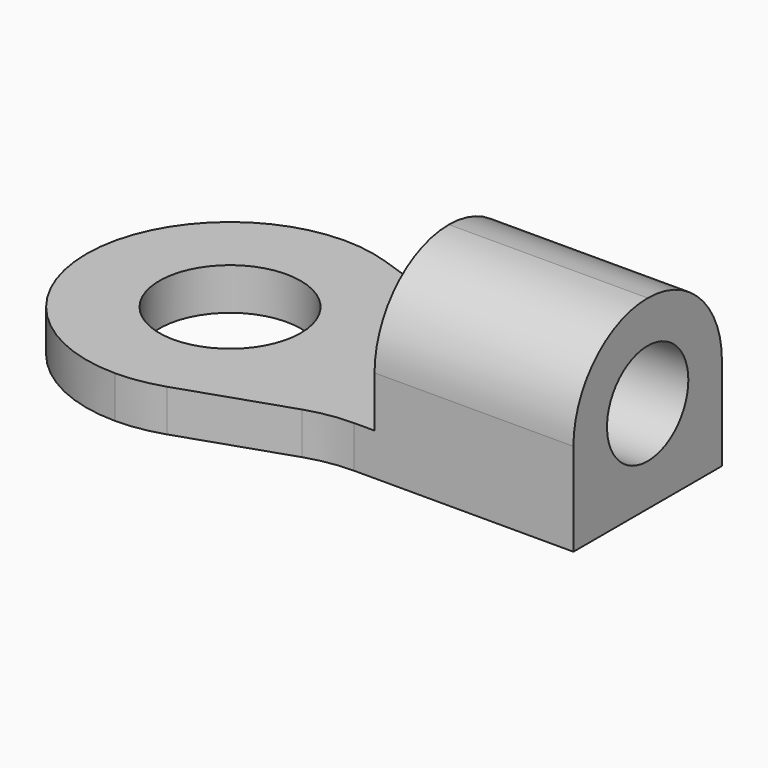
from build123d import *

# Parameters (mm, degrees)
F0_R     = 1.6
F1_DEPTH = 0.95
F2_W     = 4.5
F2_H     = 4.2
F3_DEPTH = 3.25
F4_R     = 2.09999
F5_R     = 1.15
F6_DEPTH = 25


# Not quite as in the source:
# - a fillet or chamfer is up to 0.001 mm smaller than in the source, because OpenCascade refuses the exact size


with BuildPart() as f1:
    # F0 (on Top) → F1 (new body)
    with BuildSketch(Plane.XY):
        with BuildLine():
            Line((7.7320977576, 1.15), (12.7, 1.15))
            Line((12.7, 1.15), (12.7, 5.35))
            Line((12.7, 5.35), (8.2, 5.35))
            Line((8.2, 5.35), (7.7320977576, 5.35))
            ThreePointArc((7.7320977576, 5.35), (7.2069912058, 5.3927015871), (6.6956833513, 5.5196842405))
            Line((6.6956833513, 5.5196842405), (4.2864144063, 6.3303157595))
            ThreePointArc((4.2864144063, 6.3303157595), (3.7751065518, 6.4572984129), (3.25, 6.5))
            ThreePointArc((3.25, 6.5), (0.9519029611, 5.5480970389), (0, 3.25))
            ThreePointArc((0, 3.25), (0.9519029611, 0.9519029611), (3.25, 0))
            ThreePointArc((3.25, 0), (3.7751065518, 0.0427015871), (4.2864144063, 0.1696842405))
            Line((4.2864144063, 0.1696842405), (6.6956833513, 0.9803157595))
            ThreePointArc((6.6956833513, 0.9803157595), (7.2069912058, 1.1072984129), (7.7320977576, 1.15))
        make_face()
        with Locations((3.25, 3.25)):
            Circle(F0_R, mode=Mode.SUBTRACT)
    extrude(amount=F1_DEPTH)

    # F2 (on face) → F3 (join)
    with BuildSketch(Plane.XY.offset(0.95)):
        with Locations((10.45, 3.25)):
            Rectangle(F2_W, F2_H)
    extrude(amount=F3_DEPTH)

    # F4 (radius 2.1 in the source; OpenCascade refuses exactly that, so slightly less here)
    f4_edges = [f1.edges().sort_by_distance(p)[0] for p in [
        (10.45, 5.35, 4.2),
        (10.45, 1.15, 4.2),
    ]]
    fillet(f4_edges, radius=F4_R)

    # F5 (on face) → F6 (cut)
    with BuildSketch(Plane.YZ.offset(12.7)):
        with Locations((3.25, 2.1)):
            Circle(F5_R)
    extrude(amount=-F6_DEPTH, mode=Mode.SUBTRACT)


solid = f1.part
